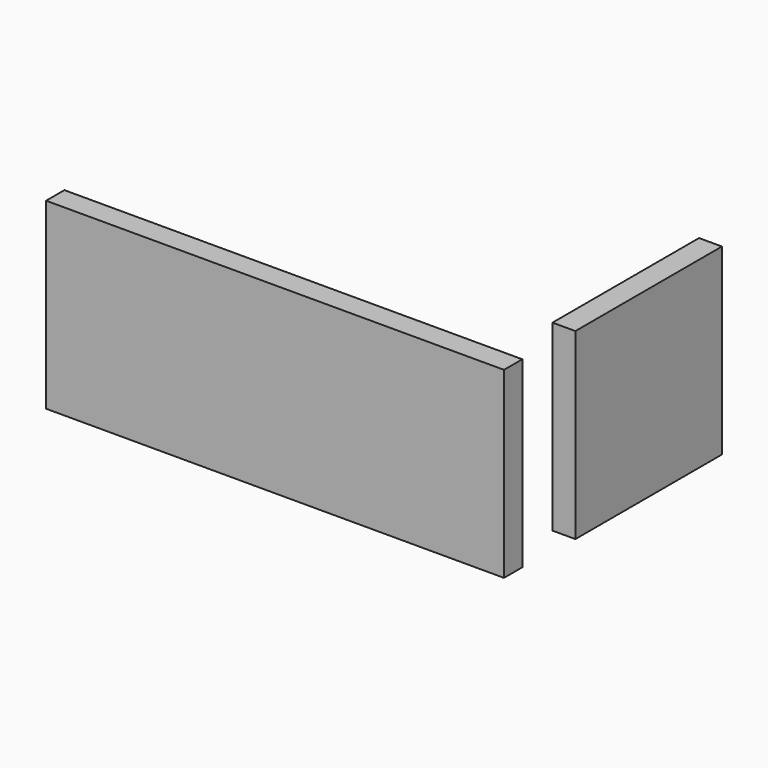
from build123d import *

# Parameters (mm, degrees)
F1_W     = 152.4
F1_H     = 152.4
F2_DEPTH = 19.05
F0_W     = 381
F0_H     = 152.4
F3_DEPTH = 19.05


# Not quite as in the source:
# - a length typed as a fraction of an inch, garbled in the dataset ("3 / 203.2 mm" for 3/8 in), is restored


with BuildPart() as f2:
    # F1 (on Right) → F2 (new body)
    with BuildSketch(Plane.YZ):
        with Locations((107.6098186895, 22.5271563627)):
            Rectangle(F1_W, F1_H)
    extrude(amount=F2_DEPTH)


with BuildPart() as f3:
    # F0 (on Front) → F3 (new body)
    with BuildSketch(Plane.XZ):
        with Locations((-190.5, 8.4438240051)):
            Rectangle(F0_W, F0_H)
    extrude(amount=F3_DEPTH)


solid = Compound([f2.part, f3.part])
